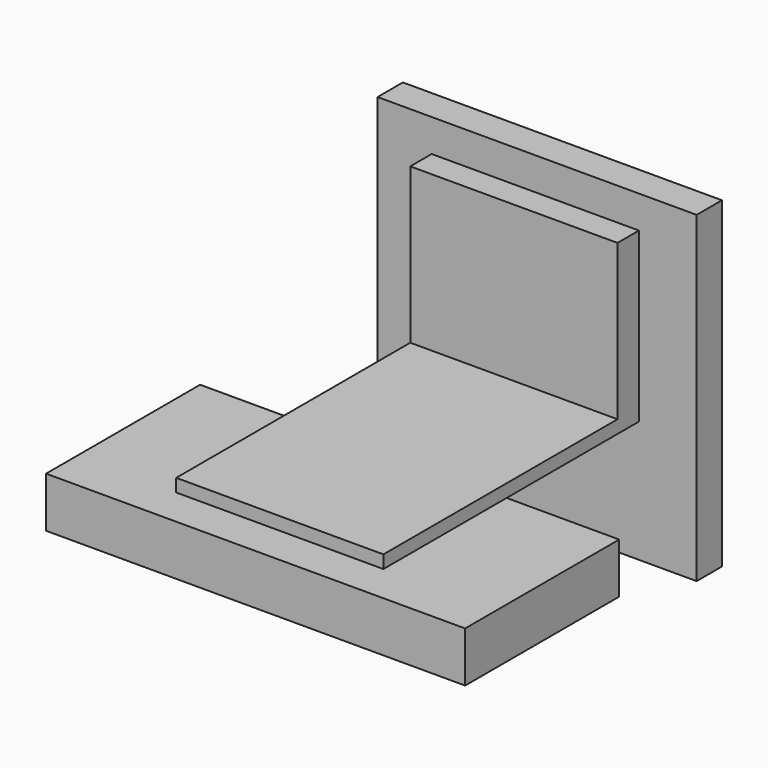
from build123d import *

# Parameters (mm, degrees)
F0_W     = 56.3671849668
F0_H     = 56.9717865437
F1_DEPTH = 5.588
F2_W     = 74.0387253463
F2_H     = 34.019369632
F3_DEPTH = 8.89
F4_W     = 36.6083486006
F4_H     = 27.2100468283
F4_H_2   = 29.2121010716
F5_DEPTH = 2.286
F6_W     = 36.6083486006
F6_H     = 4.7270159121
F7_DEPTH = 27.432


with BuildPart() as f1:
    # F0 (on Front) → F1 (new body)
    with BuildSketch(Plane.XZ):
        with Locations((6.0755070299, 6.9855386391)):
            Rectangle(F0_W, F0_H)
    extrude(amount=F1_DEPTH)


with BuildPart() as f3:
    # F2 (on Top) → F3 (new body)
    with BuildSketch(Plane.XY):
        with Locations((6.926542148, -51.8097858876)):
            Rectangle(F2_W, F2_H)
    extrude(amount=-F3_DEPTH)


with BuildPart() as f5:
    # F4 (on face) → F5 (new body)
    with BuildSketch(Plane.XY):
        with Locations((5.755436141, -48.4051244857)):
            Rectangle(F4_W, F4_H)
        with Locations((5.755436141, -20.1940505358)):
            Rectangle(F4_W, F4_H_2)
    extrude(amount=F5_DEPTH)

    # F6 (on face) → F7 (join)
    with BuildSketch(Plane.XY.offset(2.286)):
        with Locations((5.755436141, -7.951507956)):
            Rectangle(F6_W, F6_H)
    extrude(amount=F7_DEPTH)


solid = Compound([f1.part, f3.part, f5.part])
